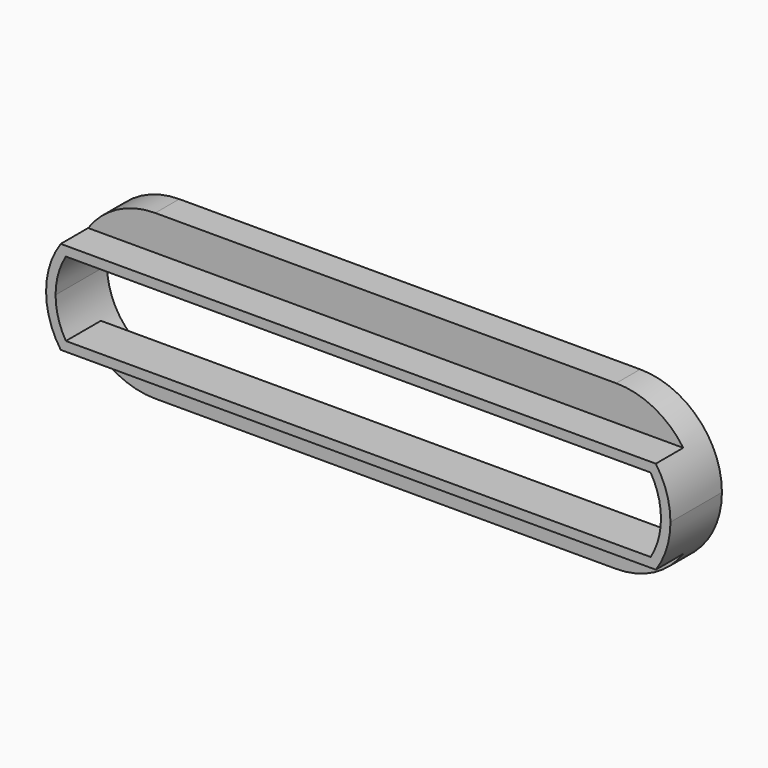
from build123d import *

# Parameters (mm, degrees)
F1_DEPTH = 5.7
F3_DEPTH = 6.5
F2_W     = 145.957624
F2_H     = 13.794057
F2_W_2   = 144.660753
F2_H_2   = 16.505709
F4_DEPTH = 25
F5_T     = -1.8


with BuildPart() as f1:
    # F0 (on Front) → F1 (new body)
    with BuildSketch(Plane.XZ):
        with BuildLine():
            Line((43.7, 15.5), (-43.7, 15.5))
            ThreePointArc((-43.7, 15.5), (-54.660155, 10.960155), (-59.2, 0))
            ThreePointArc((-59.2, 0), (-54.660155, -10.960155), (-43.7, -15.5))
            Line((-43.7, -15.5), (43.7, -15.5))
            ThreePointArc((43.7, -15.5), (54.660155, -10.960155), (59.2, 0))
            ThreePointArc((59.2, 0), (54.660155, 10.960155), (43.7, 15.5))
        make_face()
    extrude(amount=-F1_DEPTH)

    # F0 (on Front) → F3 (join)
    with BuildSketch(Plane.XZ):
        with BuildLine():
            Line((43.7, 15.5), (-43.7, 15.5))
            ThreePointArc((-43.7, 15.5), (-54.660155, 10.960155), (-59.2, 0))
            ThreePointArc((-59.2, 0), (-54.660155, -10.960155), (-43.7, -15.5))
            Line((-43.7, -15.5), (43.7, -15.5))
            ThreePointArc((43.7, -15.5), (54.660155, -10.960155), (59.2, 0))
            ThreePointArc((59.2, 0), (54.660155, 10.960155), (43.7, 15.5))
        make_face()
    extrude(amount=F3_DEPTH)

    # F2 (on Front) → F4 (cut)
    with BuildSketch(Plane.XZ):
        with Locations((-0.040472, 15.747028)):
            Rectangle(F2_W, F2_H)
        with Locations((0.372171, -17.102854)):
            Rectangle(F2_W_2, F2_H_2)
    extrude(amount=F4_DEPTH, mode=Mode.SUBTRACT)

    # F5
    f5_openings = [f1.faces().sort_by_distance(p)[0] for p in [
        (0, 5.7, 0),
        (0, -6.5, 0),
    ]]
    offset(amount=F5_T, openings=f5_openings, kind=Kind.INTERSECTION)


solid = f1.part
